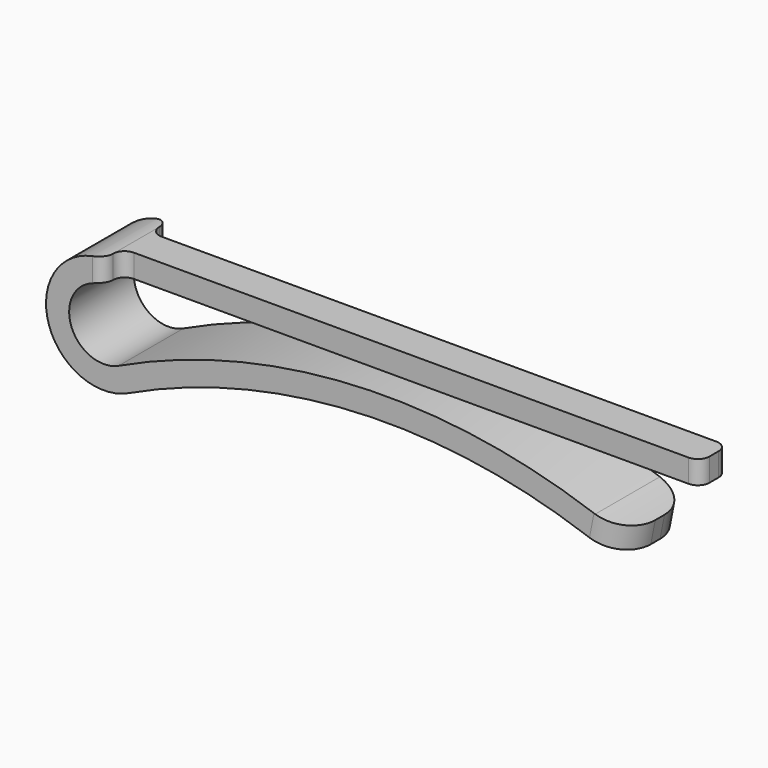
from build123d import *

# Parameters (mm, degrees)
F1_DEPTH = 7
F4_DEPTH = 2
F5_R     = 0.99999
F6_R     = 3


# Not quite as in the source:
# - a fillet or chamfer is up to 0.001 mm smaller than in the source, because OpenCascade refuses the exact size


with BuildPart() as f1:
    # F0 (on Front) → F1 (new body)
    with BuildSketch(Plane.XZ):
        with BuildLine():
            ThreePointArc((1.2846968546, -5.7110060848), (-2.9268599432, -3.6584002375), (0, 0))
            Line((0, 0), (50, 0))
            Line((50, 0), (50, 2))
            Line((50, 2), (0, 2))
            ThreePointArc((0, 2), (-4.8780999054, -4.0973337292), (2.1411614243, -7.5183434747))
            ThreePointArc((2.1411614243, -7.5183434747), (21.7926594555, -2.5678073417), (41.8462591278, -5.4905326207))
            ThreePointArc((41.8462591278, -5.4905326207), (43.3714151553, -5.9679500269), (44.9277769901, -6.3309460698))
            Line((44.9277769901, -6.3309460698), (45.3094672073, -4.3677057436))
            ThreePointArc((45.3094672073, -4.3677057436), (43.8976496677, -4.0384223028), (42.5141397524, -3.6053441762))
            ThreePointArc((42.5141397524, -3.6053441762), (21.6906488053, -0.5704105791), (1.2846968546, -5.7110060848))
        make_face()
    extrude(amount=F1_DEPTH)

    # F3 (on face) → F4 (cut)
    with BuildSketch(Plane.XY.offset(2)):
        Polygon((0, -2), (941.9215958638, -2), (50, 0), (0, 0), align=None)
        Polygon((941.9215958638, -5), (0, -5), (0, -7), (0.1395036115, -8.5481454325), (941.9215958638, -6.9726880672), align=None)
    extrude(amount=-F4_DEPTH, mode=Mode.SUBTRACT)

    # F5 (radius 1 in the source; OpenCascade refuses exactly that, so slightly less here)
    f5_edges = [f1.edges().sort_by_distance(p)[0] for p in [
        (0, 0, 1),
        (0, -5, 1),
        (50, -5, 1),
        (50, -2, 1),
        (0, -7, 1),
        (0, -2, 1),
    ]]
    fillet(f5_edges, radius=F5_R)

    # F6
    f6_edges = [f1.edges().sort_by_distance(p)[0] for p in [
        (45.118622, -7, -5.349326),
        (45.118622, 0, -5.349326),
    ]]
    fillet(f6_edges, radius=F6_R)


solid = f1.part
